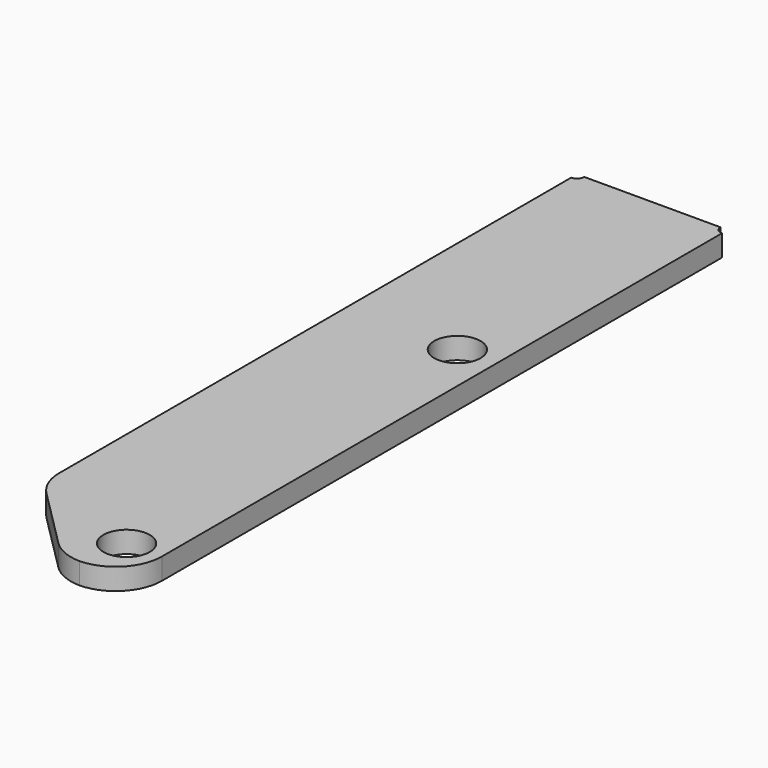
from build123d import *

# Parameters (mm, degrees)
F0_R        = 5.08
F1_DEPTH    = 4.699
F2_T1_DEPTH = 25.7410489686
F2_T3_DEPTH = 55.499


# Not quite as in the source:
# - a fillet or chamfer that OpenCascade refuses, or shapes differently, is made with other operations: its cross-section is extruded or revolved along the edge and cut away or added
# - a feature names something its author has since deleted; it is built from what else it names


with BuildPart() as f1:
    # F0 (on Top) → F1 (new body)
    with BuildSketch(Plane.XY):
        with BuildLine():
            Line((31.4325, 165.1), (1.5875, 165.1))
            ThreePointArc((1.5875, 165.1), (1.1225320151, 163.9774679849), (0, 163.5125))
            Line((0, 163.5125), (0, 19.05))
            Line((0, 19.05), (19.05, 0))
            Line((19.05, 0), (33.02, 0))
            Line((33.02, 0), (33.02, 163.5125))
            ThreePointArc((33.02, 163.5125), (31.8974679849, 163.9774679849), (31.4325, 165.1))
        make_face()
        with Locations((25.2715107054, 10.16)):
            Circle(F0_R, mode=Mode.SUBTRACT)
        with Locations((24.5934482664, 101.6)):
            Circle(F0_R, mode=Mode.SUBTRACT)
    extrude(amount=F1_DEPTH)

    # F2: fillet of radius 10.16 on 3 edges, made by hand

    # F2_s2 → F2_t1 (cut)
    with BuildSketch(Plane.XY.offset(-10.5210244843)):
        with BuildLine():
            ThreePointArc((0, 23.2584097937), (0.7733839497, 19.3703461209), (2.9757951031, 16.0742048969))
            Line((2.9757951031, 16.0742048969), (0, 19.05))
            Line((0, 19.05), (0, 23.2584097937))
        make_face()
        with BuildLine():
            ThreePointArc((16.0742048969, 2.9757951031), (19.3703461209, 0.7733839497), (23.2584097937, 0))
            Line((23.2584097937, 0), (19.05, 0))
            Line((19.05, 0), (16.0742048969, 2.9757951031))
        make_face()
    extrude(amount=F2_T1_DEPTH, mode=Mode.SUBTRACT)

    # F2_s4 → F2_t3 (cut)
    with BuildSketch(Plane.XY.offset(-25.4)):
        with BuildLine():
            ThreePointArc((22.86, 0), (30.0442048969, 2.9757951031), (33.02, 10.16))
            Line((33.02, 10.16), (33.02, 0))
            Line((33.02, 0), (22.86, 0))
        make_face()
    extrude(amount=F2_T3_DEPTH, mode=Mode.SUBTRACT)


solid = f1.part
